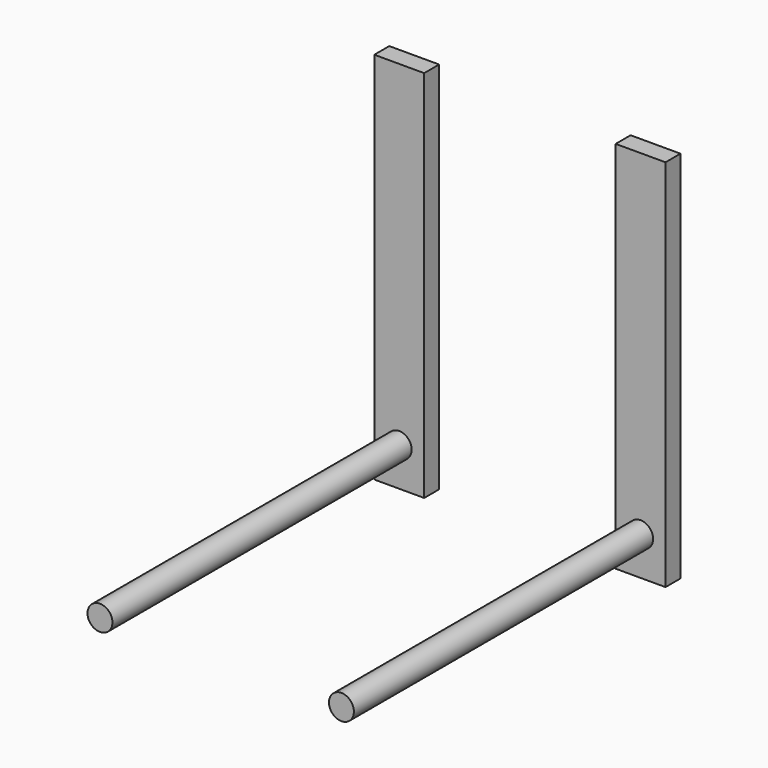
from build123d import *

# Parameters (mm, degrees)
F0_W     = 20
F0_H     = 150
F1_DEPTH = 7.5
F2_DEPTH = 7.5
F5_R     = 5
F6_DEPTH = 150


# Not quite as in the source:
# - a feature of the source that left no trace in its solid (it failed there, or was rolled back) is left out


with BuildPart() as f1:
    # F0 (on Front) → F1 (new body)
    with BuildSketch(Plane.XZ):
        with Locations((48.3931005001, -76.3607483447)):
            Rectangle(F0_W, F0_H)
    extrude(amount=F1_DEPTH)


with BuildPart() as f1b:
    # F0 (on Front) → F1, piece 2 (new body)
    with BuildSketch(Plane.XZ):
        with Locations((-48.3931005001, -76.3607483447)):
            Rectangle(F0_W, F0_H)
    extrude(amount=F1_DEPTH)


with BuildPart() as f2:
    # F2 (new): a face of the model
    f2_faces = [f1.part.faces().sort_by_distance(p)[0] for p in [
        (48.3931005001, -7.5, -76.3607483447),
    ]]
    extrude(f2_faces, amount=-F2_DEPTH)


with BuildPart() as f2b:
    # F2#2 (new): a face of the model
    f2_2_faces = [f1b.part.faces().sort_by_distance(p)[0] for p in [
        (-48.3931005001, -7.5, -76.3607483447),
    ]]
    extrude(f2_2_faces, amount=-F2_DEPTH)


with BuildPart() as f6:
    # F5 (on face) → F6 (new body)
    with BuildSketch(Plane.XZ.offset(7.5)):
        with Locations((48.4179630876, -135.9595805407)):
            Circle(F5_R)
    extrude(amount=F6_DEPTH)


with BuildPart() as f6b:
    # F5 (on face) → F6, piece 2 (new body)
    with BuildSketch(Plane.XZ.offset(7.5)):
        with Locations((-48.4179630876, -135.9595805407)):
            Circle(F5_R)
    extrude(amount=F6_DEPTH)


solid = Compound([f1.part, f1b.part, f6.part, f6b.part])
